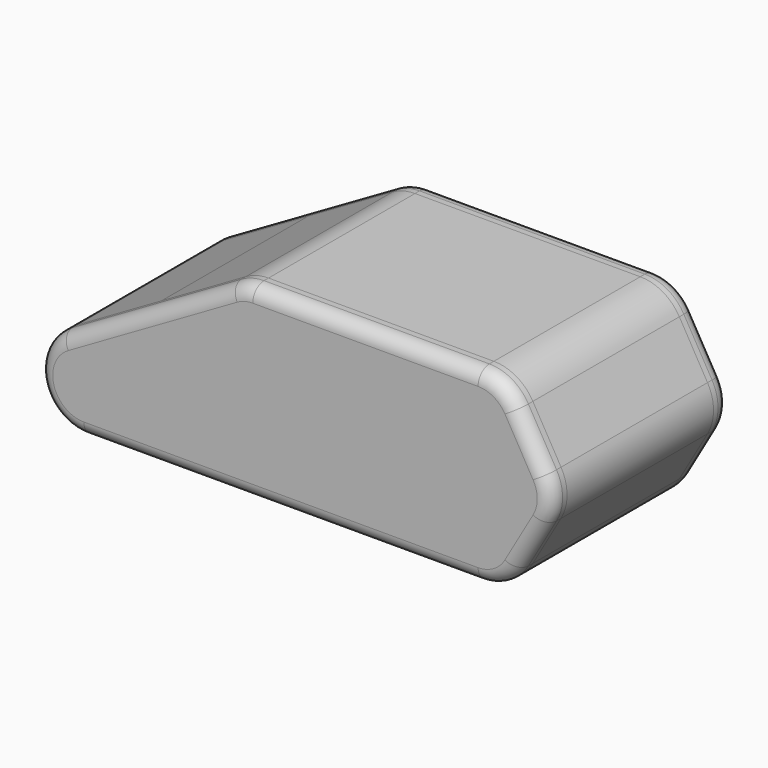
from build123d import *

# Parameters (mm, degrees)
F0_R     = 9
F1_DEPTH = 65
F2_R     = 2
F4_DEPTH = 65
F6_DEPTH = 5
F8_DEPTH = 2
F9_R     = 5
F10_R    = 4.99999


# Not quite as in the source:
# - a fillet or chamfer is up to 0.001 mm smaller than in the source, because OpenCascade refuses the exact size


with BuildPart() as f1:
    # F0 (on Front) → F1 (new body)
    with BuildSketch(Plane.XZ):
        Circle(F0_R)
    extrude(amount=F1_DEPTH)

    # F2
    f2_edges = [f1.edges().sort_by_distance(p)[0] for p in [
        (-9, 0, 0),
        (-9, -65, 0),
    ]]
    fillet(f2_edges, radius=F2_R)


with BuildPart() as f4:
    # F3 (on Front) → F4 (new body)
    with BuildSketch(Plane.XZ):
        with BuildLine():
            Line((0, -16), (140, -16))
            ThreePointArc((140, -16), (148, -13.8564064606), (153.8564064606, -8))
            Line((153.8564064606, -8), (163.8564064606, 9.3205080757))
            ThreePointArc((163.8564064606, 9.3205080757), (166, 17.3205080757), (163.8564064606, 25.3205080757))
            Line((163.8564064606, 25.3205080757), (153.8564064606, 42.6410161514))
            ThreePointArc((153.8564064606, 42.6410161514), (148, 48.4974226119), (140, 50.6410161514))
            Line((140, 50.6410161514), (60, 50.6410161514))
            ThreePointArc((60, 50.6410161514), (55.8588952784, 50.095829372), (52, 48.4974226119))
            Line((52, 48.4974226119), (22, 31.1769145362))
            Line((22, 31.1769145362), (-8, 13.8564064606))
            ThreePointArc((-8, 13.8564064606), (-15.4548132206, -4.1411047216), (0, -16))
        make_face()
        with BuildLine():
            ThreePointArc((162.124355653, 24.3205080757), (164, 17.3205080757), (162.124355653, 10.3205080757))
            Line((162.124355653, 10.3205080757), (152.124355653, -7))
            ThreePointArc((152.124355653, -7), (147, -12.124355653), (140, -14))
            Line((140, -14), (0, -14))
            ThreePointArc((0, -14), (-13.522961568, -3.6234666314), (-7, 12.124355653))
            Line((-7, 12.124355653), (23, 29.4448637287))
            Line((23, 29.4448637287), (53, 46.7653718044))
            ThreePointArc((53, 46.7653718044), (56.3765333686, 48.1639777194), (60, 48.6410161514))
            Line((60, 48.6410161514), (140, 48.6410161514))
            ThreePointArc((140, 48.6410161514), (147, 46.7653718044), (152.124355653, 41.6410161514))
            Line((152.124355653, 41.6410161514), (162.124355653, 24.3205080757))
        make_face(mode=Mode.SUBTRACT)
    extrude(amount=F4_DEPTH)


with BuildPart() as f6:
    # F5 (on face) → F6 (new body)
    with BuildSketch(Plane(origin=(0, 0, 0), x_dir=(-1, 0, 0), z_dir=(0, 1, 0))):
        with BuildLine():
            ThreePointArc((-140, 50.6410161514), (-148, 48.4974226119), (-153.8564064606, 42.6410161514))
            Line((-153.8564064606, 42.6410161514), (-163.8564064606, 25.3205080757))
            ThreePointArc((-163.8564064606, 25.3205080757), (-166, 17.3205080757), (-163.8564064606, 9.3205080757))
            Line((-163.8564064606, 9.3205080757), (-153.8564064606, -8))
            ThreePointArc((-153.8564064606, -8), (-148, -13.8564064606), (-140, -16))
            Line((-140, -16), (0, -16))
            ThreePointArc((0, -16), (15.4548132206, -4.1411047216), (8, 13.8564064606))
            Line((8, 13.8564064606), (-52, 48.4974226119))
            ThreePointArc((-52, 48.4974226119), (-55.8588952784, 50.095829372), (-60, 50.6410161514))
            Line((-60, 50.6410161514), (-140, 50.6410161514))
        make_face()
        with BuildLine():
            Line((-162.124355653, 24.3205080757), (-152.124355653, 41.6410161514))
            ThreePointArc((-152.124355653, 41.6410161514), (-147, 46.7653718044), (-140, 48.6410161514))
            Line((-140, 48.6410161514), (-60, 48.6410161514))
            ThreePointArc((-60, 48.6410161514), (-56.3765333686, 48.1639777194), (-53, 46.7653718044))
            Line((-53, 46.7653718044), (7, 12.124355653))
            ThreePointArc((7, 12.124355653), (13.522961568, -3.6234666314), (0, -14))
            Line((0, -14), (-140, -14))
            ThreePointArc((-140, -14), (-147, -12.124355653), (-152.124355653, -7))
            Line((-152.124355653, -7), (-162.124355653, 10.3205080757))
            ThreePointArc((-162.124355653, 10.3205080757), (-164, 17.3205080757), (-162.124355653, 24.3205080757))
        make_face(mode=Mode.SUBTRACT)
    extrude(amount=F6_DEPTH)

    # F7 (on face) → F8 (join)
    with BuildSketch(Plane(origin=(0, 5, 0), x_dir=(-1, 0, 0), z_dir=(0, 1, 0))):
        with BuildLine():
            Line((8, 13.8564064606), (-52, 48.4974226119))
            ThreePointArc((-52, 48.4974226119), (-55.8588952784, 50.095829372), (-60, 50.6410161514))
            Line((-60, 50.6410161514), (-140, 50.6410161514))
            ThreePointArc((-140, 50.6410161514), (-148, 48.4974226119), (-153.8564064606, 42.6410161514))
            Line((-153.8564064606, 42.6410161514), (-163.8564064606, 25.3205080757))
            ThreePointArc((-163.8564064606, 25.3205080757), (-166, 17.3205080757), (-163.8564064606, 9.3205080757))
            Line((-163.8564064606, 9.3205080757), (-153.8564064606, -8))
            ThreePointArc((-153.8564064606, -8), (-148, -13.8564064606), (-140, -16))
            Line((-140, -16), (0, -16))
            ThreePointArc((0, -16), (15.4548132206, -4.1411047216), (8, 13.8564064606))
        make_face()
        with BuildLine():
            ThreePointArc((-162.124355653, 10.3205080757), (-164, 17.3205080757), (-162.124355653, 24.3205080757))
            Line((-162.124355653, 24.3205080757), (-152.124355653, 41.6410161514))
            ThreePointArc((-152.124355653, 41.6410161514), (-147, 46.7653718044), (-140, 48.6410161514))
            Line((-140, 48.6410161514), (-60, 48.6410161514))
            ThreePointArc((-60, 48.6410161514), (-56.3765333686, 48.1639777194), (-53, 46.7653718044))
            Line((-53, 46.7653718044), (7, 12.124355653))
            ThreePointArc((7, 12.124355653), (13.522961568, -3.6234666314), (0, -14))
            Line((0, -14), (-140, -14))
            ThreePointArc((-140, -14), (-147, -12.124355653), (-152.124355653, -7))
            Line((-152.124355653, -7), (-162.124355653, 10.3205080757))
        make_face(mode=Mode.SUBTRACT)
        with BuildLine():
            Line((-152.124355653, 41.6410161514), (-162.124355653, 24.3205080757))
            ThreePointArc((-162.124355653, 24.3205080757), (-164, 17.3205080757), (-162.124355653, 10.3205080757))
            Line((-162.124355653, 10.3205080757), (-152.124355653, -7))
            ThreePointArc((-152.124355653, -7), (-147, -12.124355653), (-140, -14))
            Line((-140, -14), (0, -14))
            ThreePointArc((0, -14), (13.522961568, -3.6234666314), (7, 12.124355653))
            Line((7, 12.124355653), (-53, 46.7653718044))
            ThreePointArc((-53, 46.7653718044), (-56.3765333686, 48.1639777194), (-60, 48.6410161514))
            Line((-60, 48.6410161514), (-140, 48.6410161514))
            ThreePointArc((-140, 48.6410161514), (-147, 46.7653718044), (-152.124355653, 41.6410161514))
        make_face()
    extrude(amount=F8_DEPTH)

    # F9
    f9_edges = [f6.edges().sort_by_distance(p)[0] for p in [
        (22, 7, 31.176915),
        (55.858895, 7, 50.095829),
        (100, 7, 50.641016),
        (148, 7, 48.497423),
        (158.856406, 7, 33.980762),
        (166, 7, 17.320508),
        (158.856406, 7, 0.660254),
        (148, 7, -13.856406),
        (70, 7, -16),
        (-15.454813, 7, -4.141105),
    ]]
    fillet(f9_edges, radius=F9_R)

    # F10 (radius 5 in the source; OpenCascade refuses exactly that, so slightly less here)
    f10_edges = [f6.edges().sort_by_distance(p)[0] for p in [
        (157.124356, 5, 32.980762),
        (147, 5, 46.765372),
        (100, 5, 48.641016),
        (56.376533, 5, 48.163978),
        (23, 5, 29.444864),
        (-13.522962, 5, -3.623467),
        (70, 5, -14),
        (147, 5, -12.124356),
        (157.124356, 5, 1.660254),
        (164, 5, 17.320508),
    ]]
    fillet(f10_edges, radius=F10_R)


with BuildPart() as f12_1:
    # F12: instance of F6
    add(f6.part.mirror(Plane.XZ.offset(32.5)))


solid = Compound([f1.part, f4.part, f6.part, f12_1.part])
